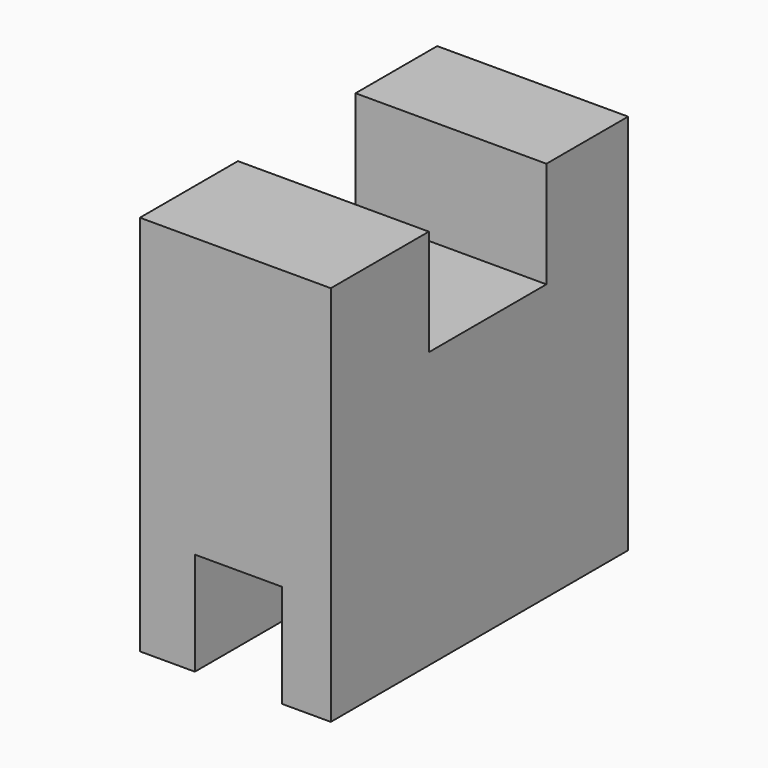
from build123d import *

# Parameters (mm, degrees)
F1_DEPTH = 12.7
F4_W     = 5.7911989279
F4_H     = 6.8580000661
F5_DEPTH = 12.7
F6_DEPTH = 25.4


# Not quite as in the source:
# - a feature of the source that left no trace in its solid (it failed there, or was rolled back) is left out


with BuildPart() as f1:
    # F0 (on Right) → F1 (new body)
    with BuildSketch(Plane.YZ):
        Polygon((12.4962570041, 25.4), (12.4962570041, 0), (37.2171103641, 0), (37.2171103641, 25.4), (30.4256705266, 25.4), (30.4256705266, 18.3368995143), (20.6459868013, 18.3368995143), (20.6459868013, 25.4), align=None)
    extrude(amount=F1_DEPTH)

    # F4 (on Front) → F5 (cut)
    with BuildSketch(Plane.XZ):
        with Locations((6.553200772, 3.4290000331)):
            Rectangle(F4_W, F4_H)
    extrude(amount=-F5_DEPTH, mode=Mode.SUBTRACT)

    # F6 (cut): a face of the model
    f6_faces = [f1.faces().sort_by_distance(p)[0] for p in [
        (6.553200772, 12.7, 3.4290000331),
    ]]
    extrude(f6_faces, amount=-F6_DEPTH, mode=Mode.SUBTRACT)


solid = f1.part
